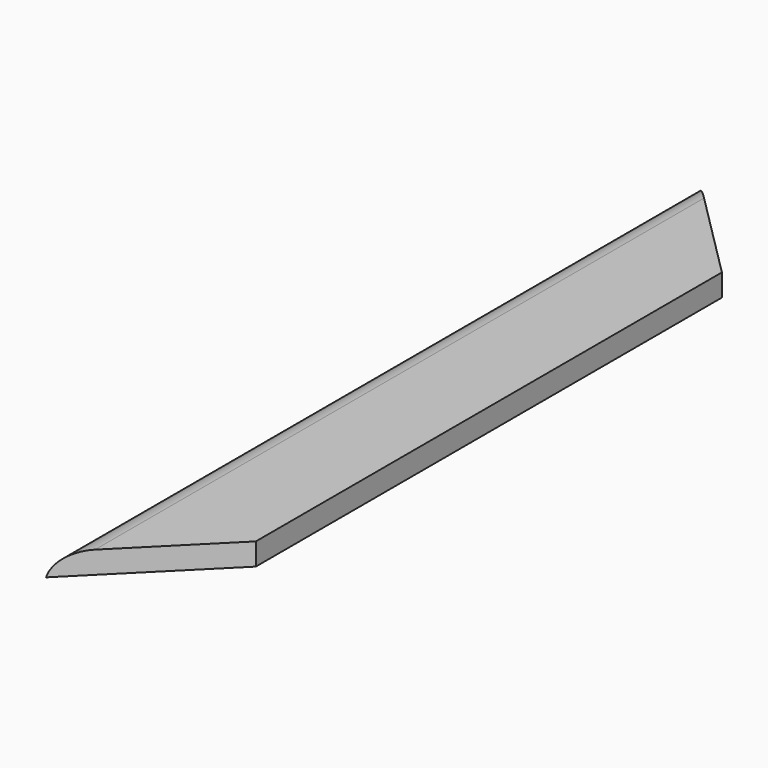
from build123d import *

# Parameters (mm, degrees)
F0_W        = 21
F0_H        = 147
F1_DEPTH    = 4
F3_DEPTH    = 4.001
F4_T1_DEPTH = 171.4948974279


# Not quite as in the source:
# - a fillet or chamfer that OpenCascade refuses, or shapes differently, is made with other operations: its cross-section is extruded or revolved along the edge and cut away or added


with BuildPart() as f1:
    # F0 (on Top) → F1 (new body)
    with BuildSketch(Plane.XY):
        Rectangle(F0_W, F0_H)
    extrude(amount=F1_DEPTH)

    # F2 (on face) → F3 (cut, through all)
    with BuildSketch(Plane.XY.offset(4)):
        Polygon((10.5, 73.5), (-10.5, 73.5), (10.5, 52.5), align=None)
        Polygon((10.5, -52.5), (-10.5, -73.5), (10.5, -73.5), align=None)
    extrude(amount=-F3_DEPTH, mode=Mode.SUBTRACT)

    # F4: fillet of radius 5 on 1 edges, made by hand

    # F4_s2 → F4_t1 (cut)
    with BuildSketch(Plane.XZ.offset(-85.7474487139)):
        with BuildLine():
            ThreePointArc((-5.6010205144, 4), (-8.7632981746, 2.8729833462), (-10.5, 0))
            Line((-10.5, 0), (-10.5, 4))
            Line((-10.5, 4), (-5.6010205144, 4))
        make_face()
    extrude(amount=F4_T1_DEPTH, mode=Mode.SUBTRACT)


solid = f1.part
